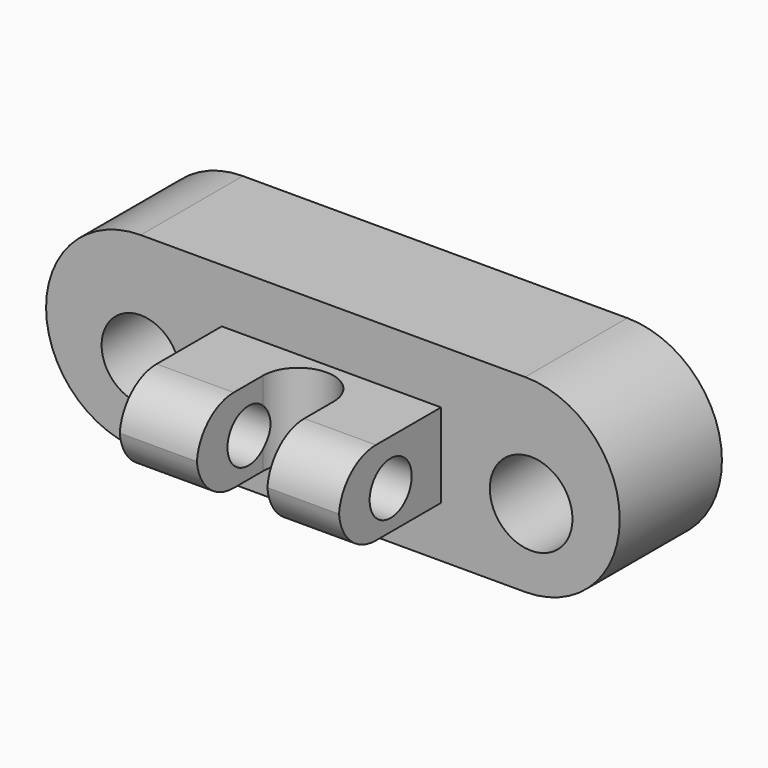
from build123d import *

# Parameters (mm, degrees)
F1_DEPTH     = 25.4
F2_R         = 7.7705666036
F2_R_2       = 8.2168581005
F3_DEPTH     = 25.4
F4_W         = 43.6024717055
F4_H         = 16.7242367752
F5_DEPTH     = 25.4
F6_R         = 5.2303111982
F7_DEPTH     = 66.548
F8_DEPTH     = 50.546
F9_W         = 14.0256546438
F9_H         = 16.4745816305
F10_DEPTH    = 27.4765354039
F11_T1_DEPTH = 61.3270374103
F11_T3_DEPTH = 60.2313163778


# Not quite as in the source:
# - a fillet or chamfer that OpenCascade refuses, or shapes differently, is made with other operations: its cross-section is extruded or revolved along the edge and cut away or added


with BuildPart() as f1:
    # F0 (on Front) → F1 (new body)
    with BuildSketch(Plane.XZ):
        with BuildLine():
            Line((53.756467998, 21.8012407422), (-22.6971805096, 21.8012407422))
            ThreePointArc((-22.6971805096, 21.8012407422), (-41.5119482204, 2.9864730313), (-22.6971805096, -15.8282946795))
            Line((-22.6971805096, -15.8282946795), (53.756467998, -15.8282946795))
            ThreePointArc((53.756467998, -15.8282946795), (72.5712357089, 2.9864730313), (53.756467998, 21.8012407422))
        make_face()
    extrude(amount=-F1_DEPTH)

    # F2 (on Front) → F3 (cut)
    with BuildSketch(Plane.XZ):
        with Locations((-22.6971805096, 0)):
            Circle(F2_R)
        with Locations((54.9510717392, 0)):
            Circle(F2_R_2)
    extrude(amount=-F3_DEPTH, mode=Mode.SUBTRACT)

    # F4 (on Front) → F5 (join)
    with BuildSketch(Plane.XZ):
        with Locations((15.2310032863, 2.6878237259)):
            Rectangle(F4_W, F4_H)
    extrude(amount=F5_DEPTH)

    # F6 (on Right) → F7 (cut)
    with BuildSketch(Plane.YZ):
        with Locations((-12.524679536, 2.001857613)):
            Circle(F6_R)
    extrude(amount=F7_DEPTH, mode=Mode.SUBTRACT)

    # F6 (on Right) → F8 (cut)
    with BuildSketch(Plane.YZ):
        with Locations((-12.524679536, 2.001857613)):
            Circle(F6_R)
    extrude(amount=-F8_DEPTH, mode=Mode.SUBTRACT)

    # F9 (on face) → F10 (cut, through all)
    with BuildSketch(Plane(origin=(0, 0, -5.6742946617), x_dir=(1, 0, 0), z_dir=(0, 0, -1))):
        with Locations((15.7788638026, 17.1627091847)):
            Rectangle(F9_W, F9_H)
        with BuildLine():
            Line((22.7916911244, 8.9254183695), (8.7660364807, 8.9254183695))
            ThreePointArc((8.7660364807, 8.9254183695), (15.7788638026, 1.9125910476), (22.7916911244, 8.9254183695))
        make_face()
    extrude(amount=-F10_DEPTH, mode=Mode.SUBTRACT)

    # F11: fillet of radius 9.1981536726 on 4 edges, made by hand

    # F11_s2 → F11_t1 (cut)
    with BuildSketch(Plane.YZ.offset(-29.565616748)):
        with BuildLine():
            ThreePointArc((-16.2018463274, -5.6742946617), (-22.7059231637, -2.9802178254), (-25.4, 3.5238590109))
            Line((-25.4, 3.5238590109), (-25.4, -5.6742946617))
            Line((-25.4, -5.6742946617), (-16.2018463274, -5.6742946617))
        make_face()
        with BuildLine():
            ThreePointArc((-16.2018463274, 11.0499421135), (-22.7059231637, 8.3558652771), (-25.4, 1.8517884408))
            Line((-25.4, 1.8517884408), (-25.4, 11.0499421135))
            Line((-25.4, 11.0499421135), (-16.2018463274, 11.0499421135))
        make_face()
    extrude(amount=F11_T1_DEPTH, mode=Mode.SUBTRACT)

    # F11_s4 → F11_t3 (cut)
    with BuildSketch(Plane.YZ.offset(-0.2036930572)):
        with BuildLine():
            ThreePointArc((-16.2018463274, -5.6742946617), (-22.7059231637, -2.9802178254), (-25.4, 3.5238590109))
            Line((-25.4, 3.5238590109), (-25.4, -5.6742946617))
            Line((-25.4, -5.6742946617), (-16.2018463274, -5.6742946617))
        make_face()
        with BuildLine():
            ThreePointArc((-16.2018463274, 11.0499421135), (-22.7059231637, 8.3558652771), (-25.4, 1.8517884408))
            Line((-25.4, 1.8517884408), (-25.4, 11.0499421135))
            Line((-25.4, 11.0499421135), (-16.2018463274, 11.0499421135))
        make_face()
    extrude(amount=F11_T3_DEPTH, mode=Mode.SUBTRACT)


solid = f1.part
